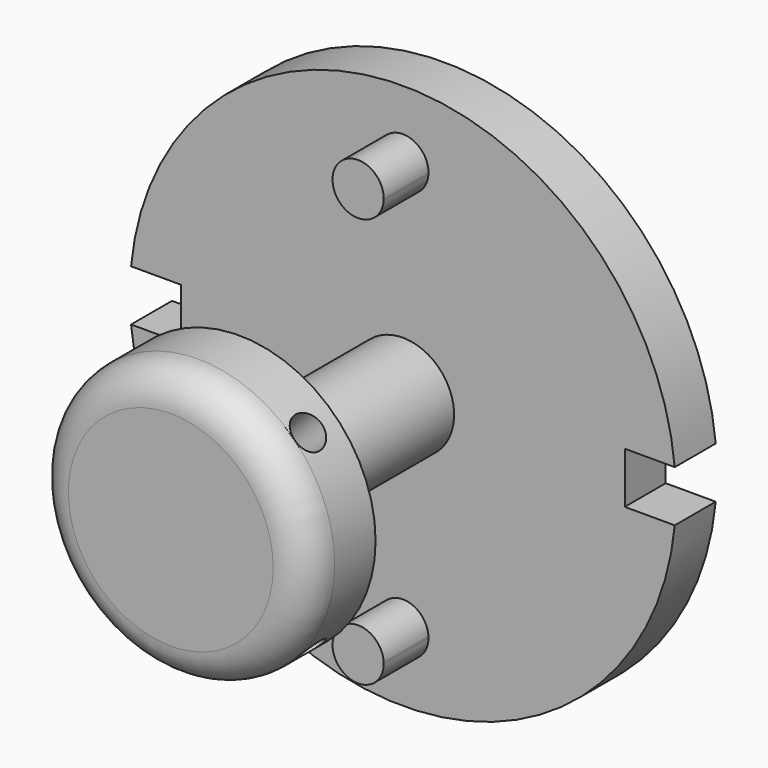
from build123d import *

# Parameters (mm, degrees)
F1_DEPTH  = 19.05
F2_DEPTH  = 76.2
F3_DEPTH  = 20.828
F4_DEPTH  = 38.1
F5_DEPTH  = 63.5
F6_R      = 50.8
F6_R_2    = 19.05
F7_DEPTH  = 31.75
F8_R      = 12.7
F19_D     = 12.7
F19_DEPTH = 16.002
F19_START = 0.3984376
F19_TIP   = 3.8154649308
F20_D     = 12.7
F20_DEPTH = 16.002
F20_START = 0.3984376
F20_TIP   = 3.8154649308
F21_D     = 12.7
F21_DEPTH = 16.002
F21_START = 0.3984376
F21_TIP   = 3.8154649308
F22_D     = 12.7
F22_DEPTH = 16.002
F22_START = 0.3984376
F22_TIP   = 3.8154649308


with BuildPart() as f1:
    # F0 (on Front) → F1 (new body)
    with BuildSketch(Plane.XZ):
        with BuildLine():
            Line((82.55, 9.525), (101.1525302452, 9.525))
            ThreePointArc((101.1525302452, 9.525), (0, 101.6), (-101.1525302452, 9.525))
            Line((-101.1525302452, 9.525), (-82.55, 9.525))
            Line((-82.55, 9.525), (-82.55, 0))
            Line((-82.55, 0), (-76.2, 0))
            ThreePointArc((-76.2, 0), (-57.1437924233, 50.4086003325), (-9.5063782813, 75.6046875))
            ThreePointArc((-9.5063782813, 75.6046875), (-0.2978018389, 85.7203434321), (9.525, 76.2))
            ThreePointArc((9.525, 76.2), (9.5203434321, 75.9021981611), (9.5063782813, 75.6046875))
            ThreePointArc((9.5063782813, 75.6046875), (57.1437924233, 50.4086003325), (76.2, 0))
            Line((76.2, 0), (82.55, 0))
            Line((82.55, 0), (82.55, 9.525))
        make_face()
        with BuildLine():
            ThreePointArc((-101.1525302452, -9.525), (0, -101.6), (101.1525302452, -9.525))
            Line((101.1525302452, -9.525), (82.55, -9.525))
            Line((82.55, -9.525), (82.55, 0))
            Line((82.55, 0), (76.2, 0))
            ThreePointArc((76.2, 0), (57.1437924233, -50.4086003325), (9.5063782813, -75.6046875))
            ThreePointArc((9.5063782813, -75.6046875), (9.5203434321, -75.9021981611), (9.525, -76.2))
            ThreePointArc((9.525, -76.2), (-0.2978018389, -85.7203434321), (-9.5063782813, -75.6046875))
            ThreePointArc((-9.5063782813, -75.6046875), (-57.1437924233, -50.4086003325), (-76.2, 0))
            Line((-76.2, 0), (-82.55, 0))
            Line((-82.55, 0), (-82.55, -9.525))
            Line((-82.55, -9.525), (-101.1525302452, -9.525))
        make_face()
        with BuildLine():
            ThreePointArc((9.5063782813, -75.6046875), (57.1437924233, -50.4086003325), (76.2, 0))
            Line((76.2, 0), (50.8, 0))
            ThreePointArc((50.8, 0), (0, -50.8), (-50.8, 0))
            Line((-50.8, 0), (-76.2, 0))
            ThreePointArc((-76.2, 0), (-57.1437924233, -50.4086003325), (-9.5063782813, -75.6046875))
            ThreePointArc((-9.5063782813, -75.6046875), (0, -66.675), (9.5063782813, -75.6046875))
        make_face()
        with BuildLine():
            ThreePointArc((-50.8, 0), (0, -50.8), (50.8, 0))
            Line((50.8, 0), (25.4, 0))
            ThreePointArc((25.4, 0), (0, -25.4), (-25.4, 0))
            Line((-25.4, 0), (-50.8, 0))
        make_face()
        with BuildLine():
            Line((25.4, 0), (50.8, 0))
            ThreePointArc((50.8, 0), (0, 50.8), (-50.8, 0))
            Line((-50.8, 0), (-25.4, 0))
            ThreePointArc((-25.4, 0), (0, 25.4), (25.4, 0))
        make_face()
        with BuildLine():
            Line((50.8, 0), (76.2, 0))
            ThreePointArc((76.2, 0), (57.1437924233, 50.4086003325), (9.5063782813, 75.6046875))
            ThreePointArc((9.5063782813, 75.6046875), (0, 66.675), (-9.5063782813, 75.6046875))
            ThreePointArc((-9.5063782813, 75.6046875), (-57.1437924233, 50.4086003325), (-76.2, 0))
            Line((-76.2, 0), (-50.8, 0))
            ThreePointArc((-50.8, 0), (0, 50.8), (50.8, 0))
        make_face()
        with BuildLine():
            ThreePointArc((-19.05, 0), (0, -19.05), (19.05, 0))
            Line((19.05, 0), (0, 0))
            Line((0, 0), (-19.05, 0))
        make_face()
        with BuildLine():
            Line((0, 0), (19.05, 0))
            ThreePointArc((19.05, 0), (0, 19.05), (-19.05, 0))
            Line((-19.05, 0), (0, 0))
        make_face()
        with BuildLine():
            ThreePointArc((9.525, -76.2), (9.5203434321, -75.9021981611), (9.5063782813, -75.6046875))
            ThreePointArc((9.5063782813, -75.6046875), (0, -76.2), (-9.5063782813, -75.6046875))
            ThreePointArc((-9.5063782813, -75.6046875), (-0.2978018389, -85.7203434321), (9.525, -76.2))
        make_face()
        with BuildLine():
            ThreePointArc((-9.5063782813, 75.6046875), (0, 66.675), (9.5063782813, 75.6046875))
            ThreePointArc((9.5063782813, 75.6046875), (0, 76.2), (-9.5063782813, 75.6046875))
        make_face()
        with BuildLine():
            ThreePointArc((-9.5063782813, 75.6046875), (0, 76.2), (9.5063782813, 75.6046875))
            ThreePointArc((9.5063782813, 75.6046875), (9.5203434321, 75.9021981611), (9.525, 76.2))
            ThreePointArc((9.525, 76.2), (-0.2978018389, 85.7203434321), (-9.5063782813, 75.6046875))
        make_face()
        with BuildLine():
            ThreePointArc((-9.5063782813, -75.6046875), (0, -76.2), (9.5063782813, -75.6046875))
            ThreePointArc((9.5063782813, -75.6046875), (0, -66.675), (-9.5063782813, -75.6046875))
        make_face()
        with BuildLine():
            ThreePointArc((-25.4, 0), (0, -25.4), (25.4, 0))
            Line((25.4, 0), (19.05, 0))
            ThreePointArc((19.05, 0), (0, -19.05), (-19.05, 0))
            Line((-19.05, 0), (-25.4, 0))
        make_face()
        with BuildLine():
            Line((19.05, 0), (25.4, 0))
            ThreePointArc((25.4, 0), (0, 25.4), (-25.4, 0))
            Line((-25.4, 0), (-19.05, 0))
            ThreePointArc((-19.05, 0), (0, 19.05), (19.05, 0))
        make_face()
    extrude(amount=-F1_DEPTH)

    # F0 (on Front) → F2 (join)
    with BuildSketch(Plane.XZ):
        with BuildLine():
            Line((0, 0), (19.05, 0))
            ThreePointArc((19.05, 0), (0, 19.05), (-19.05, 0))
            Line((-19.05, 0), (0, 0))
        make_face()
        with BuildLine():
            ThreePointArc((-19.05, 0), (0, -19.05), (19.05, 0))
            Line((19.05, 0), (0, 0))
            Line((0, 0), (-19.05, 0))
        make_face()
    extrude(amount=F2_DEPTH)

    # F0 (on Front) → F3 (join)
    with BuildSketch(Plane.XZ):
        with BuildLine():
            ThreePointArc((-9.5063782813, -75.6046875), (0, -76.2), (9.5063782813, -75.6046875))
            ThreePointArc((9.5063782813, -75.6046875), (0, -66.675), (-9.5063782813, -75.6046875))
        make_face()
        with BuildLine():
            ThreePointArc((9.525, -76.2), (9.5203434321, -75.9021981611), (9.5063782813, -75.6046875))
            ThreePointArc((9.5063782813, -75.6046875), (0, -76.2), (-9.5063782813, -75.6046875))
            ThreePointArc((-9.5063782813, -75.6046875), (-0.2978018389, -85.7203434321), (9.525, -76.2))
        make_face()
        with BuildLine():
            ThreePointArc((-9.5063782813, 75.6046875), (0, 66.675), (9.5063782813, 75.6046875))
            ThreePointArc((9.5063782813, 75.6046875), (0, 76.2), (-9.5063782813, 75.6046875))
        make_face()
        with BuildLine():
            ThreePointArc((-9.5063782813, 75.6046875), (0, 76.2), (9.5063782813, 75.6046875))
            ThreePointArc((9.5063782813, 75.6046875), (9.5203434321, 75.9021981611), (9.525, 76.2))
            ThreePointArc((9.525, 76.2), (-0.2978018389, 85.7203434321), (-9.5063782813, 75.6046875))
        make_face()
    extrude(amount=F3_DEPTH)

    # F0 (on Front) → F4 (join)
    with BuildSketch(Plane.XZ):
        with BuildLine():
            Line((19.05, 0), (25.4, 0))
            ThreePointArc((25.4, 0), (0, 25.4), (-25.4, 0))
            Line((-25.4, 0), (-19.05, 0))
            ThreePointArc((-19.05, 0), (0, 19.05), (19.05, 0))
        make_face()
        with BuildLine():
            ThreePointArc((-25.4, 0), (0, -25.4), (25.4, 0))
            Line((25.4, 0), (19.05, 0))
            ThreePointArc((19.05, 0), (0, -19.05), (-19.05, 0))
            Line((-19.05, 0), (-25.4, 0))
        make_face()
    extrude(amount=-F4_DEPTH)

    # F5 (add): a face of the model
    f5_faces = [f1.faces().sort_by_distance(p)[0] for p in [
        (0, 19.05, 0),
    ]]
    extrude(f5_faces, amount=F5_DEPTH)

    # F6 (on face) → F7 (join)
    with BuildSketch(Plane.XZ.offset(76.2)):
        Circle(F6_R)
        Circle(F6_R_2, mode=Mode.SUBTRACT)
        Circle(F6_R_2)
    extrude(amount=F7_DEPTH)

    # F8
    f8_edges = [f1.edges().sort_by_distance(p)[0] for p in [
        (-50.8, -107.95, 0),
    ]]
    fillet(f8_edges, radius=F8_R)

    # F19
    # its depths count from where the whole tool has entered the part; down to there all is cleared
    with Locations(Plane(origin=(35.9210244843, 0, -35.9210244843), x_dir=(0.7071067812, 0, 0.7071067812), z_dir=(0.7071067812, 0, -0.7071067812)).offset(-F19_START)):
        with Locations((0, 88.9)):
            Hole(F19_D / 2, depth=F19_DEPTH)
            with Locations((0, 0, -(F19_DEPTH + F19_TIP / 2))):  # 118° drill point
                Cone(0, F19_D / 2, F19_TIP, mode=Mode.SUBTRACT)

    # F20
    # its depths count from where the whole tool has entered the part; down to there all is cleared
    with Locations(Plane(origin=(-35.9210244843, 0, -35.9210244843), x_dir=(0, -1, 0), z_dir=(-0.7071067812, 0, -0.7071067812)).offset(-F20_START)):
        with Locations((88.9, 0)):
            Hole(F20_D / 2, depth=F20_DEPTH)
            with Locations((0, 0, -(F20_DEPTH + F20_TIP / 2))):  # 118° drill point
                Cone(0, F20_D / 2, F20_TIP, mode=Mode.SUBTRACT)

    # F21
    # its depths count from where the whole tool has entered the part; down to there all is cleared
    with Locations(Plane(origin=(35.9210244843, 0, 35.9210244843), x_dir=(0, -1, 0), z_dir=(0.7071067812, 0, 0.7071067812)).offset(-F21_START)):
        with Locations((88.9, 0)):
            Hole(F21_D / 2, depth=F21_DEPTH)
            with Locations((0, 0, -(F21_DEPTH + F21_TIP / 2))):  # 118° drill point
                Cone(0, F21_D / 2, F21_TIP, mode=Mode.SUBTRACT)

    # F22
    # its depths count from where the whole tool has entered the part; down to there all is cleared
    with Locations(Plane(origin=(-35.9210244843, 0, 35.9210244843), x_dir=(0.7071067812, 0, 0.7071067812), z_dir=(-0.7071067812, 0, 0.7071067812)).offset(-F22_START)):
        with Locations((0, -88.9)):
            Hole(F22_D / 2, depth=F22_DEPTH)
            with Locations((0, 0, -(F22_DEPTH + F22_TIP / 2))):  # 118° drill point
                Cone(0, F22_D / 2, F22_TIP, mode=Mode.SUBTRACT)


solid = f1.part
